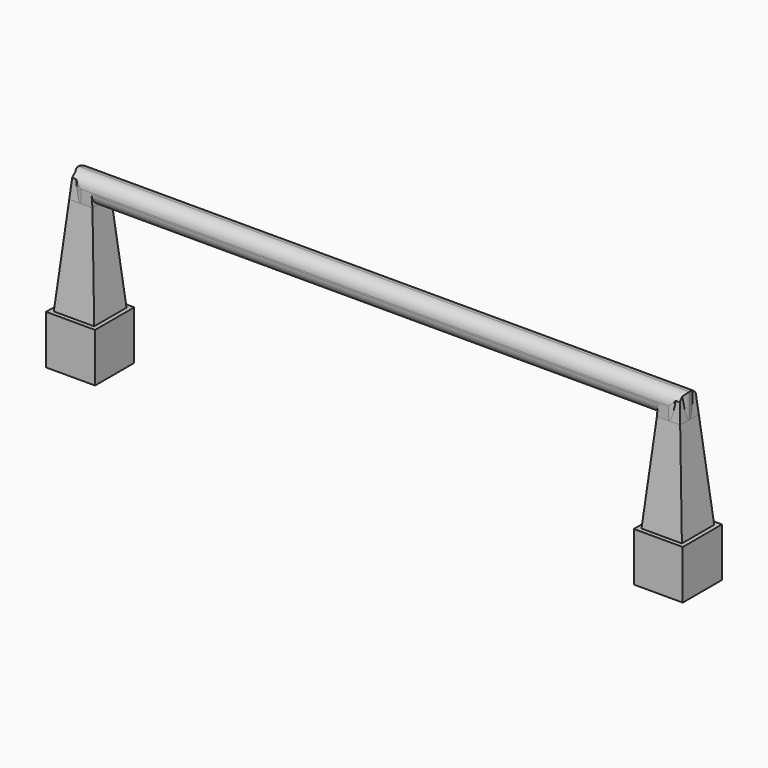
from build123d import *

# Parameters (mm, degrees)
F0_W         = 5
F0_H         = 5
F1_DEPTH     = 5
F2_DEPTH     = 15
F2_TAPER     = 5
F4_DEPTH     = 2.5
F5_T4_DEPTH  = 8.4
F5_T9_DEPTH  = 8.4
F5_T14_DEPTH = 8.4
F5_T19_DEPTH = 8.4
F5_T24_DEPTH = 8.4
F5_T29_DEPTH = 8.4
F5_T34_DEPTH = 8.4
F5_T39_DEPTH = 8.4
F6_T1_DEPTH  = 65.9153400942
F6_T6_DEPTH  = 63.5246599058
F6_T12_DEPTH = 63.5246599058


# Not quite as in the source:
# - a fillet or chamfer that OpenCascade refuses, or shapes differently, is made with other operations: its cross-section is extruded or revolved along the edge and cut away or added


with BuildPart() as f1:
    # F0 (on Top) → F1 (new body)
    with BuildSketch(Plane.XY):
        with Locations((-2.5, 2.5)):
            Rectangle(F0_W, F0_H)
    extrude(amount=F1_DEPTH)

    # F0 (on Top) → F2 (join)
    with BuildSketch(Plane.XY):
        with Locations((-2.5, 2.5)):
            Rectangle(F0_W, F0_H)
    extrude(amount=F2_DEPTH, taper=F2_TAPER)



with BuildPart() as f1b:
    # F0 (on Top) → F1, piece 2 (new body)
    with BuildSketch(Plane.XY):
        with Locations((57.5, 2.5)):
            Rectangle(F0_W, F0_H)
    extrude(amount=F1_DEPTH)

    # F0 (on Top) → F2, piece 2 (join)
    with BuildSketch(Plane.XY):
        with Locations((57.5, 2.5)):
            Rectangle(F0_W, F0_H)
    extrude(amount=F2_DEPTH, taper=F2_TAPER)


with BuildPart() as f1_1:
    add(f1.part)

    add(f1b.part)  # F4 merges F1b
    # F3 (on face) → F4 (join)
    with BuildSketch(Plane.XY.offset(15)):
        Polygon((-1.3123299529, 3.6876700471), (-3.6876700471, 3.6876700471), (-3.6876700471, 1.3123299529), (-1.3123299529, 1.3123299529), (56.3123299529, 1.3123299529), (58.6876700471, 1.3123299529), (58.6876700471, 3.6876700471), (56.3123299529, 3.6876700471), align=None)
    extrude(amount=F4_DEPTH)

    # F5: fillet of radius 1.18 on 4 edges, made by hand


with BuildPart() as f5_tool2:
    # F5_s3 → F5_t4 (new body)
    with BuildSketch(Plane.XY.offset(12.05)):
        with BuildLine():
            ThreePointArc((58.6876700471, 2.5076700471), (58.3420560489, 3.3420560489), (57.5076700471, 3.6876700471))
            Line((57.5076700471, 3.6876700471), (58.6876700471, 3.6876700471))
            Line((58.6876700471, 3.6876700471), (58.6876700471, 2.5076700471))
        make_face()
    extrude(amount=F5_T4_DEPTH)

    split(bisect_by=Plane(origin=(0, 4.9620193825, 0.4341204442), x_dir=(1, 0, 0), z_dir=(0, 0.9961946981, 0.0871557427)), keep=Keep.TOP)


with BuildPart() as f1_2:
    add(f1_1.part)

    # F5_t1: cut F5_tool2
    add(f5_tool2.part, mode=Mode.SUBTRACT)


with BuildPart() as f5_tool7:
    # F5_s8 → F5_t9 (new body)
    with BuildSketch(Plane.XY.offset(12.05)):
        with BuildLine():
            ThreePointArc((58.6876700471, 2.5076700471), (58.3420560489, 3.3420560489), (57.5076700471, 3.6876700471))
            Line((57.5076700471, 3.6876700471), (58.6876700471, 3.6876700471))
            Line((58.6876700471, 3.6876700471), (58.6876700471, 2.5076700471))
        make_face()
    extrude(amount=F5_T9_DEPTH)

    split(bisect_by=Plane(origin=(59.5442325904, 0, 5.20944533), x_dir=(0, 1, 0), z_dir=(0.9961946981, 0, 0.0871557427)), keep=Keep.TOP)


with BuildPart() as f1_3:
    add(f1_2.part)

    # F5_t6: cut F5_tool7
    add(f5_tool7.part, mode=Mode.SUBTRACT)


with BuildPart() as f5_tool12:
    # F5_s13 → F5_t14 (new body)
    with BuildSketch(Plane.XY.offset(12.05)):
        with BuildLine():
            ThreePointArc((57.5076700471, 1.3123299529), (58.3420560489, 1.6579439511), (58.6876700471, 2.4923299529))
            Line((58.6876700471, 2.4923299529), (58.6876700471, 1.3123299529))
            Line((58.6876700471, 1.3123299529), (57.5076700471, 1.3123299529))
        make_face()
    extrude(amount=F5_T14_DEPTH)

    split(bisect_by=Plane(origin=(59.5442325904, 0, 5.20944533), x_dir=(0, 1, 0), z_dir=(0.9961946981, 0, 0.0871557427)), keep=Keep.TOP)


with BuildPart() as f1_4:
    add(f1_3.part)

    # F5_t11: cut F5_tool12
    add(f5_tool12.part, mode=Mode.SUBTRACT)


with BuildPart() as f5_tool17:
    # F5_s18 → F5_t19 (new body)
    with BuildSketch(Plane.XY.offset(12.05)):
        with BuildLine():
            ThreePointArc((57.5076700471, 1.3123299529), (58.3420560489, 1.6579439511), (58.6876700471, 2.4923299529))
            Line((58.6876700471, 2.4923299529), (58.6876700471, 1.3123299529))
            Line((58.6876700471, 1.3123299529), (57.5076700471, 1.3123299529))
        make_face()
    extrude(amount=F5_T19_DEPTH)

    split(bisect_by=Plane(origin=(0, 0, 0), x_dir=(1, 0, 0), z_dir=(0, -0.9961946981, 0.0871557427)), keep=Keep.TOP)


with BuildPart() as f1_5:
    add(f1_4.part)

    # F5_t16: cut F5_tool17
    add(f5_tool17.part, mode=Mode.SUBTRACT)


with BuildPart() as f5_tool22:
    # F5_s23 → F5_t24 (new body)
    with BuildSketch(Plane.XY.offset(12.05)):
        with BuildLine():
            ThreePointArc((-2.5076700471, 3.6876700471), (-3.3420560489, 3.3420560489), (-3.6876700471, 2.5076700471))
            Line((-3.6876700471, 2.5076700471), (-3.6876700471, 3.6876700471))
            Line((-3.6876700471, 3.6876700471), (-2.5076700471, 3.6876700471))
        make_face()
    extrude(amount=F5_T24_DEPTH)

    split(bisect_by=Plane(origin=(-4.9620193825, 0, 0.4341204442), x_dir=(0, 1, 0), z_dir=(-0.9961946981, 0, 0.0871557427)), keep=Keep.TOP)


with BuildPart() as f1_6:
    add(f1_5.part)

    # F5_t21: cut F5_tool22
    add(f5_tool22.part, mode=Mode.SUBTRACT)


with BuildPart() as f5_tool27:
    # F5_s28 → F5_t29 (new body)
    with BuildSketch(Plane.XY.offset(12.05)):
        with BuildLine():
            ThreePointArc((-2.5076700471, 3.6876700471), (-3.3420560489, 3.3420560489), (-3.6876700471, 2.5076700471))
            Line((-3.6876700471, 2.5076700471), (-3.6876700471, 3.6876700471))
            Line((-3.6876700471, 3.6876700471), (-2.5076700471, 3.6876700471))
        make_face()
    extrude(amount=F5_T29_DEPTH)

    split(bisect_by=Plane(origin=(0, 4.9620193825, 0.4341204442), x_dir=(1, 0, 0), z_dir=(0, 0.9961946981, 0.0871557427)), keep=Keep.TOP)


with BuildPart() as f1_7:
    add(f1_6.part)

    # F5_t26: cut F5_tool27
    add(f5_tool27.part, mode=Mode.SUBTRACT)


with BuildPart() as f5_tool32:
    # F5_s33 → F5_t34 (new body)
    with BuildSketch(Plane.XY.offset(12.05)):
        with BuildLine():
            ThreePointArc((-2.5076700471, 1.3123299529), (-3.3420560489, 1.6579439511), (-3.6876700471, 2.4923299529))
            Line((-3.6876700471, 2.4923299529), (-3.6876700471, 1.3123299529))
            Line((-3.6876700471, 1.3123299529), (-2.5076700471, 1.3123299529))
        make_face()
    extrude(amount=F5_T34_DEPTH)

    split(bisect_by=Plane(origin=(-4.9620193825, 0, 0.4341204442), x_dir=(0, 1, 0), z_dir=(-0.9961946981, 0, 0.0871557427)), keep=Keep.TOP)


with BuildPart() as f1_8:
    add(f1_7.part)

    # F5_t31: cut F5_tool32
    add(f5_tool32.part, mode=Mode.SUBTRACT)


with BuildPart() as f5_tool37:
    # F5_s38 → F5_t39 (new body)
    with BuildSketch(Plane.XY.offset(12.05)):
        with BuildLine():
            ThreePointArc((-2.5076700471, 1.3123299529), (-3.3420560489, 1.6579439511), (-3.6876700471, 2.4923299529))
            Line((-3.6876700471, 2.4923299529), (-3.6876700471, 1.3123299529))
            Line((-3.6876700471, 1.3123299529), (-2.5076700471, 1.3123299529))
        make_face()
    extrude(amount=F5_T39_DEPTH)

    split(bisect_by=Plane(origin=(0, 0, 0), x_dir=(1, 0, 0), z_dir=(0, -0.9961946981, 0.0871557427)), keep=Keep.TOP)


with BuildPart() as f1_9:
    add(f1_8.part)

    # F5_t36: cut F5_tool37
    add(f5_tool37.part, mode=Mode.SUBTRACT)

    # F6: fillet of radius 1.18 on 8 edges, made by hand

    # F6_s2 → F6_t1 (cut)
    with BuildSketch(Plane.YZ.offset(-5.4576700471)):
        with BuildLine():
            ThreePointArc((3.6876700471, 16.32), (3.3420560489, 17.1543860018), (2.5076700471, 17.5))
            Line((2.5076700471, 17.5), (3.6876700471, 17.5))
            Line((3.6876700471, 17.5), (3.6876700471, 16.32))
        make_face()
        with BuildLine():
            ThreePointArc((2.4923299529, 17.5), (1.6579439511, 17.1543860018), (1.3123299529, 16.32))
            Line((1.3123299529, 16.32), (1.3123299529, 17.5))
            Line((1.3123299529, 17.5), (2.4923299529, 17.5))
        make_face()
    extrude(amount=F6_T1_DEPTH, mode=Mode.SUBTRACT)


with BuildPart() as f6_tool4:
    # F6_s5 → F6_t6 (new body)
    with BuildSketch(Plane.YZ.offset(59.2623299529)):
        with BuildLine():
            ThreePointArc((2.5076700471, 15), (3.3420560489, 15.3456139982), (3.6876700471, 16.18))
            Line((3.6876700471, 16.18), (3.6876700471, 15))
            Line((3.6876700471, 15), (2.5076700471, 15))
        make_face()
    extrude(amount=-F6_T6_DEPTH)

    split(bisect_by=Plane(origin=(54.5822132078, 0, -4.7753248858), x_dir=(0, 1, 0), z_dir=(-0.9961946981, 0, 0.0871557427)), keep=Keep.TOP)

    split(bisect_by=Plane(origin=(0, 0, 0), x_dir=(0, 1, 0), z_dir=(0.9961946981, 0, 0.0871557427)), keep=Keep.TOP)


with BuildPart() as f1_10:
    add(f1_9.part)

    # F6_t3: cut F6_tool4
    add(f6_tool4.part, mode=Mode.SUBTRACT)


with BuildPart() as f6_tool10:
    # F6_s11 → F6_t12 (new body)
    with BuildSketch(Plane.YZ.offset(-4.2623299529)):
        with BuildLine():
            ThreePointArc((2.4923299529, 15), (1.6579439511, 15.3456139982), (1.3123299529, 16.18))
            Line((1.3123299529, 16.18), (1.3123299529, 15))
            Line((1.3123299529, 15), (2.4923299529, 15))
        make_face()
    extrude(amount=F6_T12_DEPTH)

    split(bisect_by=Plane(origin=(54.5822132078, 0, -4.7753248858), x_dir=(0, 1, 0), z_dir=(-0.9961946981, 0, 0.0871557427)), keep=Keep.TOP)

    split(bisect_by=Plane(origin=(0, 0, 0), x_dir=(0, 1, 0), z_dir=(0.9961946981, 0, 0.0871557427)), keep=Keep.TOP)


with BuildPart() as f1_11:
    add(f1_10.part)

    # F6_t9: cut F6_tool10
    add(f6_tool10.part, mode=Mode.SUBTRACT)


solid = f1_11.part
